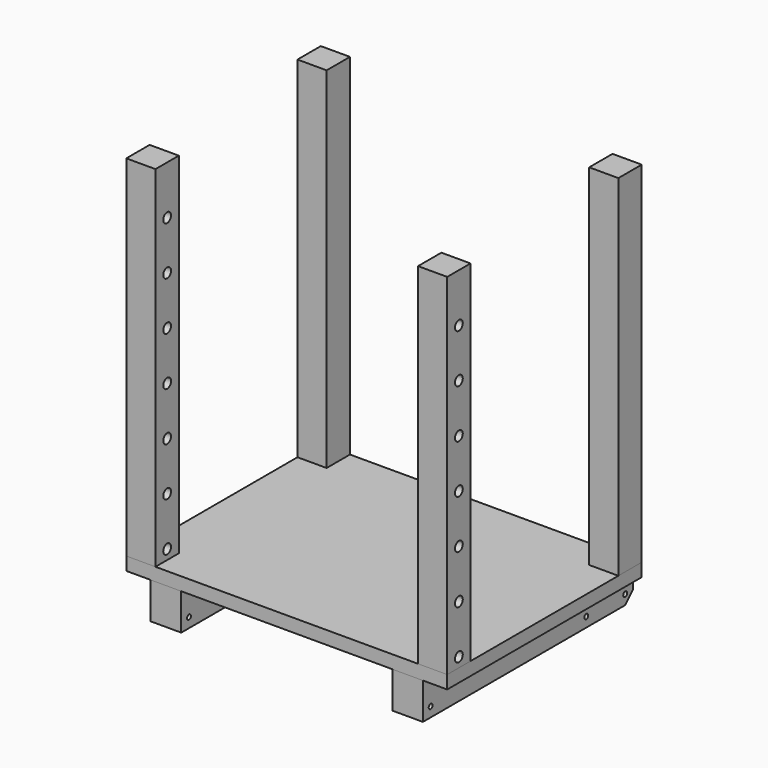
from build123d import *

# Parameters (mm, degrees)
F0_W      = 660
F0_H      = 500
F1_DEPTH  = 27
F2_W      = 60
F2_H      = 60
F3_DEPTH  = 720
F4_W      = 63
F4_H      = 63
F4_H_2    = 40
F4_H_3    = 33
F5_DEPTH  = 75
F6_R      = 5
F7_DEPTH  = 610.001
F9_R      = 5
F10_DEPTH = 610.001
F12_DEPTH = 610.001
F8_R      = 10
F13_DEPTH = 660.001


# Not quite as in the source:
# - a feature names something its author has since deleted; it is built from what else it names


with BuildPart() as f1:
    # F0 (on Top) → F1 (new body)
    with BuildSketch(Plane.XY):
        Rectangle(F0_W, F0_H)
    extrude(amount=F1_DEPTH)


with BuildPart() as f3:
    # F2 (on face) → F3 (new body)
    with BuildSketch(Plane.XY.offset(27)):
        with Locations((-300, 220)):
            Rectangle(F2_W, F2_H)
    extrude(amount=F3_DEPTH)


with BuildPart() as f3b:
    # F2 (on face) → F3, piece 2 (new body)
    with BuildSketch(Plane.XY.offset(27)):
        with Locations((300, 220)):
            Rectangle(F2_W, F2_H)
    extrude(amount=F3_DEPTH)


with BuildPart() as f3c:
    # F2 (on face) → F3, piece 3 (new body)
    with BuildSketch(Plane.XY.offset(27)):
        with Locations((300, -220)):
            Rectangle(F2_W, F2_H)
    extrude(amount=F3_DEPTH)


with BuildPart() as f3d:
    # F2 (on face) → F3, piece 4 (new body)
    with BuildSketch(Plane.XY.offset(27)):
        with Locations((-300, -220)):
            Rectangle(F2_W, F2_H)
    extrude(amount=F3_DEPTH)


with BuildPart() as f5:
    # F4 (on face) → F5 (new body)
    with BuildSketch(Plane(origin=(0, 0, 0), x_dir=(1, 0, 0), z_dir=(0, 0, -1))):
        with Locations((-248.5, -218.5)):
            Rectangle(F4_W, F4_H)
        with Locations((-248.5, -270)):
            Rectangle(F4_W, F4_H_2)
        Polygon((-280, 217), (-280, -154), (-217, -154), (-217, 217), (-217, 250), (-280, 250), align=None)
        with Locations((-248.5, -170.5)):
            Rectangle(F4_W, F4_H_3)
    extrude(amount=F5_DEPTH)


with BuildPart() as f5b:
    # F4 (on face) → F5, piece 2 (new body)
    with BuildSketch(Plane(origin=(0, 0, 0), x_dir=(1, 0, 0), z_dir=(0, 0, -1))):
        with Locations((248.5, -270)):
            Rectangle(F4_W, F4_H_2)
        with Locations((248.5, -218.5)):
            Rectangle(F4_W, F4_H)
        Polygon((217, 217), (217, -154), (280, -154), (280, 217), (280, 250), (217, 250), align=None)
        with Locations((248.5, -170.5)):
            Rectangle(F4_W, F4_H_3)
    extrude(amount=F5_DEPTH)


with BuildPart() as f7_tool:
    # F6 (on face) → F7 (new body, through all)
    with BuildSketch(Plane(origin=(-280, 0, 0), x_dir=(0, -1, 0), z_dir=(-1, 0, 0))):
        with Locations((-270, -55)):
            Circle(F6_R)
    extrude(amount=-F7_DEPTH)


with BuildPart() as f5_1:
    add(f5.part)

    # F7: cut by f7_tool
    add(f7_tool.part, mode=Mode.SUBTRACT)


with BuildPart() as f5b_1:
    add(f5b.part)

    # F7: cut by f7_tool
    add(f7_tool.part, mode=Mode.SUBTRACT)


with BuildPart() as f10_tool:
    # F9 (on face) → F10 (new body, through all)
    with BuildSketch(Plane(origin=(-280, 0, 0), x_dir=(0, -1, 0), z_dir=(-1, 0, 0))):
        with Locations((230, -55)):
            Circle(F9_R)
        with Locations((-170, -55)):
            Circle(F9_R)
    extrude(amount=-F10_DEPTH)


with BuildPart() as f5_2:
    add(f5_1.part)

    # F10: cut by f10_tool
    add(f10_tool.part, mode=Mode.SUBTRACT)


with BuildPart() as f5b_2:
    add(f5b_1.part)

    # F10: cut by f10_tool
    add(f10_tool.part, mode=Mode.SUBTRACT)


with BuildPart() as f12_tool:
    # F11 (on face) → F12 (new body, through all)
    with BuildSketch(Plane(origin=(-280, 0, 0), x_dir=(0, -1, 0), z_dir=(-1, 0, 0))):
        Polygon((-290, -55), (-290, -75), (-270, -75), align=None)
    extrude(amount=-F12_DEPTH)


with BuildPart() as f5_3:
    add(f5_2.part)

    # F12: cut by f12_tool
    add(f12_tool.part, mode=Mode.SUBTRACT)


with BuildPart() as f5b_3:
    add(f5b_2.part)

    # F12: cut by f12_tool
    add(f12_tool.part, mode=Mode.SUBTRACT)


with BuildPart() as f13_tool:
    # F8 (on face) → F13 (new body, through all)
    with BuildSketch(Plane(origin=(-330, 0, 0), x_dir=(0, -1, 0), z_dir=(-1, 0, 0))):
        with Locations((220, 647)):
            Circle(F8_R)
        with Locations((220, 547)):
            Circle(F8_R)
        with Locations((220, 447)):
            Circle(F8_R)
        with Locations((220, 347)):
            Circle(F8_R)
        with Locations((220, 247)):
            Circle(F8_R)
        with Locations((-220, 647)):
            Circle(F8_R)
        with Locations((-220, 547)):
            Circle(F8_R)
        with Locations((-220, 447)):
            Circle(F8_R)
        with Locations((-220, 347)):
            Circle(F8_R)
        with Locations((-220, 247)):
            Circle(F8_R)
        with Locations((-220, 147)):
            Circle(F8_R)
        with Locations((-220, 47)):
            Circle(F8_R)
        with Locations((220, 147)):
            Circle(F8_R)
        with Locations((220, 47)):
            Circle(F8_R)
    extrude(amount=-F13_DEPTH)


with BuildPart() as f3c_1:
    add(f3c.part)

    # F13: cut by f13_tool
    add(f13_tool.part, mode=Mode.SUBTRACT)


with BuildPart() as f3d_1:
    add(f3d.part)

    # F13: cut by f13_tool
    add(f13_tool.part, mode=Mode.SUBTRACT)


solid = Compound([f1.part, f3.part, f3b.part, f5_3.part, f5b_3.part, f3c_1.part, f3d_1.part])
